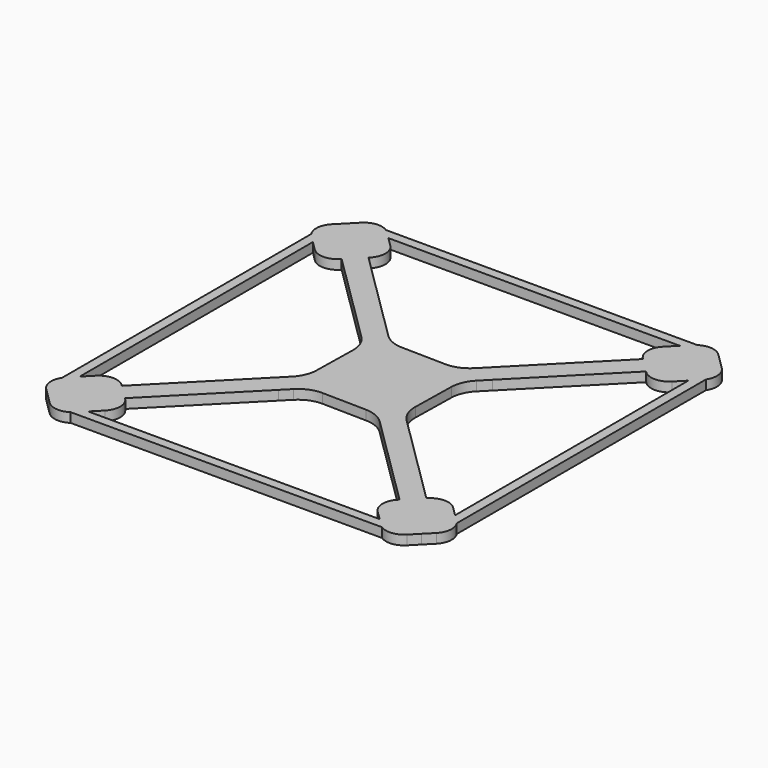
from build123d import *

# Parameters (mm, degrees)
F1_DEPTH = 4
F3_DEPTH = 4


with BuildPart() as f1:
    # F0 (on Top) → F1 (new body)
    with BuildSketch(Plane.XY):
        with BuildLine():
            Line((-64.135030253, 57.8487346722), (-60.9918824626, 60.9918824626))
            Line((-60.9918824626, 60.9918824626), (-57.8872043507, 64.1730347516))
            Line((-57.8872043507, 64.1730347516), (-57.5279368508, 64.536699731))
            ThreePointArc((-57.5279368508, 64.536699731), (-55.3289064598, 69.9383294266), (-57.5934861455, 75.3128077153))
            Line((-57.5934861455, 75.3128077153), (-61.0650929383, 78.7424354322))
            Line((-61.0650929383, 78.7424354322), (-64.536699731, 82.1720631491))
            ThreePointArc((-64.536699731, 82.1720631491), (-69.9383294266, 84.3710935402), (-75.3128077153, 82.1065138545))
            Line((-75.3128077153, 82.1065138545), (-78.7424354322, 78.6349070617))
            Line((-78.7424354322, 78.6349070617), (-82.1720631491, 75.163300269))
            ThreePointArc((-82.1720631491, 75.163300269), (-84.3710935402, 69.7616705734), (-82.1065138545, 64.3871922846))
            Line((-82.1065138545, 64.3871922846), (-75.163300269, 57.5279368508))
            ThreePointArc((-75.163300269, 57.5279368508), (-69.7616705734, 55.3289064598), (-64.3871922846, 57.5934861455))
            Line((-64.3871922846, 57.5934861455), (-64.135030253, 57.8487346722))
        make_face()
        with BuildLine():
            Line((-60.9918824626, 60.9918824626), (-24.9487193947, 24.9487193947))
            ThreePointArc((-24.9487193947, 24.9487193947), (-23.2982405477, 26.6622275187), (-21.7131078047, 28.4363596169))
            Line((-21.7131078047, 28.4363596169), (-57.8872043507, 64.1730347516))
            Line((-57.8872043507, 64.1730347516), (-60.9918824626, 60.9918824626))
        make_face()
        with BuildLine():
            ThreePointArc((-27.9685415263, 22.1195753621), (-26.4355788417, 23.5095421312), (-24.9487193947, 24.9487193947))
            Line((-24.9487193947, 24.9487193947), (-60.9918824626, 60.9918824626))
            Line((-60.9918824626, 60.9918824626), (-64.135030253, 57.8487346722))
            Line((-64.135030253, 57.8487346722), (-27.9685415263, 22.1195753621))
        make_face()
        with BuildLine():
            Line((-24.9487193947, 24.9487193947), (0, 0))
            Line((0, 0), (24.9487193947, 24.9487193947))
            ThreePointArc((24.9487193947, 24.9487193947), (23.5095421312, 26.4355788417), (22.1195753621, 27.9685415263))
            Line((22.1195753621, 27.9685415263), (18.6042693789, 24.4102077544))
            ThreePointArc((18.6042693789, 24.4102077544), (14.3526979396, 21.5708297932), (9.3259920152, 20.6380090919))
            Line((9.3259920152, 20.6380090919), (-9.2049935755, 20.9934651587))
            ThreePointArc((-9.2049935755, 20.9934651587), (-13.8982384325, 21.9899359298), (-17.8868961856, 24.6564149968))
            Line((-17.8868961856, 24.6564149968), (-21.7131078047, 28.4363596169))
            ThreePointArc((-21.7131078047, 28.4363596169), (-23.2982405477, 26.6622275187), (-24.9487193947, 24.9487193947))
        make_face()
        with BuildLine():
            Line((-24.6564149968, -17.8868961856), (-28.4363596169, -21.7131078047))
            ThreePointArc((-28.4363596169, -21.7131078047), (-26.6622275187, -23.2982405478), (-24.9487193947, -24.9487193947))
            Line((-24.9487193947, -24.9487193947), (0, 0))
            Line((0, 0), (-24.9487193947, 24.9487193947))
            ThreePointArc((-24.9487193947, 24.9487193947), (-26.4355788417, 23.5095421312), (-27.9685415263, 22.1195753621))
            Line((-27.9685415263, 22.1195753621), (-24.4102077544, 18.6042693789))
            ThreePointArc((-24.4102077544, 18.6042693789), (-21.5708297932, 14.3526979396), (-20.6380090919, 9.3259920152))
            Line((-20.6380090919, 9.3259920152), (-20.9934651587, -9.2049935755))
            ThreePointArc((-20.9934651587, -9.2049935755), (-21.9899359298, -13.8982384325), (-24.6564149968, -17.8868961856))
        make_face()
        with BuildLine():
            ThreePointArc((-24.9487193947, -24.9487193947), (-23.5095421312, -26.4355788418), (-22.1195753621, -27.9685415263))
            Line((-22.1195753621, -27.9685415263), (-18.6042693789, -24.4102077545))
            ThreePointArc((-18.6042693789, -24.4102077545), (-14.3526979396, -21.5708297932), (-9.3259920152, -20.6380090919))
            Line((-9.3259920152, -20.6380090919), (9.2049935755, -20.9934651587))
            ThreePointArc((9.2049935755, -20.9934651587), (13.8982384325, -21.9899359298), (17.8868961856, -24.6564149968))
            Line((17.8868961856, -24.6564149968), (21.7131078047, -28.4363596169))
            ThreePointArc((21.7131078047, -28.4363596169), (23.2982405477, -26.6622275187), (24.9487193947, -24.9487193947))
            Line((24.9487193947, -24.9487193947), (0, 0))
            Line((0, 0), (-24.9487193947, -24.9487193947))
        make_face()
        with BuildLine():
            Line((24.9487193947, 24.9487193947), (0, 0))
            Line((0, 0), (24.9487193947, -24.9487193947))
            ThreePointArc((24.9487193947, -24.9487193947), (26.4355788417, -23.5095421312), (27.9685415263, -22.1195753621))
            Line((27.9685415263, -22.1195753621), (24.4102077545, -18.6042693789))
            ThreePointArc((24.4102077545, -18.6042693789), (21.5708297932, -14.3526979396), (20.6380090919, -9.3259920152))
            Line((20.6380090919, -9.3259920152), (20.9934651587, 9.2049935755))
            ThreePointArc((20.9934651587, 9.2049935755), (21.9899359298, 13.8982384325), (24.6564149968, 17.8868961856))
            Line((24.6564149968, 17.8868961856), (28.4363596169, 21.7131078047))
            ThreePointArc((28.4363596169, 21.7131078047), (26.6622275187, 23.2982405477), (24.9487193947, 24.9487193947))
        make_face()
        with BuildLine():
            Line((60.9918824626, 60.9918824626), (24.9487193947, 24.9487193947))
            ThreePointArc((24.9487193947, 24.9487193947), (26.6622275187, 23.2982405477), (28.4363596169, 21.7131078047))
            Line((28.4363596169, 21.7131078047), (64.1730347516, 57.8872043507))
            Line((64.1730347516, 57.8872043507), (60.9918824626, 60.9918824626))
        make_face()
        with BuildLine():
            ThreePointArc((22.1195753621, 27.9685415263), (23.5095421312, 26.4355788417), (24.9487193947, 24.9487193947))
            Line((24.9487193947, 24.9487193947), (60.9918824626, 60.9918824626))
            Line((60.9918824626, 60.9918824626), (57.8487346722, 64.135030253))
            Line((57.8487346722, 64.135030253), (22.1195753621, 27.9685415263))
        make_face()
        with BuildLine():
            Line((57.8487346722, 64.135030253), (60.9918824626, 60.9918824626))
            Line((60.9918824626, 60.9918824626), (64.1730347516, 57.8872043507))
            Line((64.1730347516, 57.8872043507), (64.536699731, 57.5279368508))
            ThreePointArc((64.536699731, 57.5279368508), (69.9383294266, 55.3289064598), (75.3128077154, 57.5934861455))
            Line((75.3128077154, 57.5934861455), (78.7424354323, 61.0650929383))
            Line((78.7424354323, 61.0650929383), (82.1720631492, 64.536699731))
            ThreePointArc((82.1720631492, 64.536699731), (84.3710935402, 69.9383294266), (82.1065138545, 75.3128077153))
            Line((82.1065138545, 75.3128077153), (78.6349070617, 78.7424354322))
            Line((78.6349070617, 78.7424354322), (75.163300269, 82.1720631491))
            ThreePointArc((75.163300269, 82.1720631491), (69.7616705734, 84.3710935402), (64.3871922846, 82.1065138545))
            Line((64.3871922846, 82.1065138545), (57.5279368508, 75.163300269))
            ThreePointArc((57.5279368508, 75.163300269), (55.3289064598, 69.7616705734), (57.5934861455, 64.3871922846))
            Line((57.5934861455, 64.3871922846), (57.8487346722, 64.135030253))
        make_face()
        with BuildLine():
            Line((64.135030253, -57.8487346722), (60.9918824626, -60.9918824626))
            Line((60.9918824626, -60.9918824626), (57.8872043507, -64.1730347516))
            Line((57.8872043507, -64.1730347516), (57.5279368509, -64.536699731))
            ThreePointArc((57.5279368509, -64.536699731), (55.3289064598, -69.9383294266), (57.5934861455, -75.3128077154))
            Line((57.5934861455, -75.3128077154), (61.0650929383, -78.7424354323))
            Line((61.0650929383, -78.7424354323), (64.536699731, -82.1720631492))
            ThreePointArc((64.536699731, -82.1720631492), (69.9383294266, -84.3710935402), (75.3128077154, -82.1065138545))
            Line((75.3128077154, -82.1065138545), (78.7424354323, -78.6349070617))
            Line((78.7424354323, -78.6349070617), (82.1720631492, -75.163300269))
            ThreePointArc((82.1720631492, -75.163300269), (84.3710935402, -69.7616705734), (82.1065138545, -64.3871922846))
            Line((82.1065138545, -64.3871922846), (75.163300269, -57.5279368508))
            ThreePointArc((75.163300269, -57.5279368508), (69.7616705734, -55.3289064598), (64.3871922847, -57.5934861455))
            Line((64.3871922847, -57.5934861455), (64.135030253, -57.8487346722))
        make_face()
        with BuildLine():
            ThreePointArc((27.9685415263, -22.1195753621), (26.4355788417, -23.5095421312), (24.9487193947, -24.9487193947))
            Line((24.9487193947, -24.9487193947), (60.9918824626, -60.9918824626))
            Line((60.9918824626, -60.9918824626), (64.135030253, -57.8487346722))
            Line((64.135030253, -57.8487346722), (27.9685415263, -22.1195753621))
        make_face()
        with BuildLine():
            Line((60.9918824626, -60.9918824626), (24.9487193947, -24.9487193947))
            ThreePointArc((24.9487193947, -24.9487193947), (23.2982405477, -26.6622275187), (21.7131078047, -28.4363596169))
            Line((21.7131078047, -28.4363596169), (57.8872043507, -64.1730347516))
            Line((57.8872043507, -64.1730347516), (60.9918824626, -60.9918824626))
        make_face()
        with BuildLine():
            Line((-57.8487346722, -64.135030253), (-22.1195753621, -27.9685415263))
            ThreePointArc((-22.1195753621, -27.9685415263), (-23.5095421312, -26.4355788418), (-24.9487193947, -24.9487193947))
            Line((-24.9487193947, -24.9487193947), (-60.9918824626, -60.9918824626))
            Line((-60.9918824626, -60.9918824626), (-57.8487346722, -64.135030253))
        make_face()
        with BuildLine():
            ThreePointArc((-24.9487193947, -24.9487193947), (-26.6622275187, -23.2982405478), (-28.4363596169, -21.7131078047))
            Line((-28.4363596169, -21.7131078047), (-64.1730347516, -57.8872043507))
            Line((-64.1730347516, -57.8872043507), (-60.9918824626, -60.9918824626))
            Line((-60.9918824626, -60.9918824626), (-24.9487193947, -24.9487193947))
        make_face()
        with BuildLine():
            Line((-57.5934861455, -64.3871922847), (-57.8487346722, -64.135030253))
            Line((-57.8487346722, -64.135030253), (-60.9918824626, -60.9918824626))
            Line((-60.9918824626, -60.9918824626), (-64.1730347516, -57.8872043507))
            Line((-64.1730347516, -57.8872043507), (-64.536699731, -57.5279368509))
            ThreePointArc((-64.536699731, -57.5279368509), (-69.9383294266, -55.3289064598), (-75.3128077153, -57.5934861455))
            Line((-75.3128077153, -57.5934861455), (-78.7424354322, -61.0650929383))
            Line((-78.7424354322, -61.0650929383), (-82.1720631491, -64.536699731))
            ThreePointArc((-82.1720631491, -64.536699731), (-84.3710935402, -69.9383294266), (-82.1065138545, -75.3128077154))
            Line((-82.1065138545, -75.3128077154), (-78.6349070617, -78.7424354323))
            Line((-78.6349070617, -78.7424354323), (-75.163300269, -82.1720631492))
            ThreePointArc((-75.163300269, -82.1720631492), (-69.7616705734, -84.3710935402), (-64.3871922846, -82.1065138545))
            Line((-64.3871922846, -82.1065138545), (-57.5279368508, -75.163300269))
            ThreePointArc((-57.5279368508, -75.163300269), (-55.3289064598, -69.7616705734), (-57.5934861455, -64.3871922847))
        make_face()
    extrude(amount=F1_DEPTH)

    # F2 (on face) → F3 (join)
    with BuildSketch(Plane.XY.offset(4)):
        with BuildLine():
            ThreePointArc((-64.3871922846, -82.1065138545), (-64.9658566006, -82.634927624), (-65.5957303462, -83.1011170351))
            Line((-65.5957303462, -83.1011170351), (65.6796884979, -83.1011170351))
            ThreePointArc((65.6796884979, -83.1011170351), (65.0856932086, -82.6642723213), (64.536699731, -82.1720631492))
            Line((64.536699731, -82.1720631492), (61.4281648492, -79.1011170351))
            Line((61.4281648492, -79.1011170351), (-61.4181370755, -79.1011170351))
            Line((-61.4181370755, -79.1011170351), (-64.3871922846, -82.1065138545))
        make_face()
        with BuildLine():
            ThreePointArc((-75.163300269, -82.1720631492), (-70.5444929949, -84.335561038), (-65.5957303462, -83.1011170351))
            ThreePointArc((-65.5957303462, -83.1011170351), (-64.9658566006, -82.634927624), (-64.3871922846, -82.1065138545))
            Line((-64.3871922846, -82.1065138545), (-61.4181370755, -79.1011170351))
            Line((-61.4181370755, -79.1011170351), (-57.5279368508, -75.163300269))
            ThreePointArc((-57.5279368508, -75.163300269), (-55.3289064598, -69.7616705734), (-57.5934861455, -64.3871922847))
            Line((-57.5934861455, -64.3871922847), (-57.8487346722, -64.135030253))
            Line((-57.8487346722, -64.135030253), (-18.6042693789, -24.4102077545))
            ThreePointArc((-18.6042693789, -24.4102077545), (-14.3526979396, -21.5708297932), (-9.3259920152, -20.6380090919))
            Line((-9.3259920152, -20.6380090919), (9.2049935755, -20.9934651587))
            ThreePointArc((9.2049935755, -20.9934651587), (13.8982384325, -21.9899359298), (17.8868961856, -24.6564149968))
            Line((17.8868961856, -24.6564149968), (57.8872043507, -64.1730347516))
            Line((57.8872043507, -64.1730347516), (57.5279368509, -64.536699731))
            ThreePointArc((57.5279368509, -64.536699731), (55.3289064598, -69.9383294266), (57.5934861455, -75.3128077154))
            Line((57.5934861455, -75.3128077154), (61.4281648492, -79.1011170351))
            Line((61.4281648492, -79.1011170351), (64.536699731, -82.1720631492))
            ThreePointArc((64.536699731, -82.1720631492), (65.0856932086, -82.6642723213), (65.6796884979, -83.1011170351))
            ThreePointArc((65.6796884979, -83.1011170351), (70.6745708809, -84.3309409727), (75.3128077154, -82.1065138545))
            Line((75.3128077154, -82.1065138545), (82.1720631492, -75.163300269))
            ThreePointArc((82.1720631492, -75.163300269), (84.335561038, -70.5444929949), (83.1011170351, -65.5957303462))
            ThreePointArc((83.1011170351, -65.5957303462), (82.634927624, -64.9658566006), (82.1065138545, -64.3871922846))
            Line((82.1065138545, -64.3871922846), (79.1011170351, -61.4181370755))
            Line((79.1011170351, -61.4181370755), (75.163300269, -57.5279368508))
            ThreePointArc((75.163300269, -57.5279368508), (69.7616705734, -55.3289064598), (64.3871922847, -57.5934861455))
            Line((64.3871922847, -57.5934861455), (64.135030253, -57.8487346722))
            Line((64.135030253, -57.8487346722), (24.4102077545, -18.6042693789))
            ThreePointArc((24.4102077545, -18.6042693789), (21.5708297932, -14.3526979396), (20.6380090919, -9.3259920152))
            Line((20.6380090919, -9.3259920152), (20.9934651587, 9.2049935755))
            ThreePointArc((20.9934651587, 9.2049935755), (21.9899359298, 13.8982384325), (24.6564149968, 17.8868961856))
            Line((24.6564149968, 17.8868961856), (64.1730347516, 57.8872043507))
            Line((64.1730347516, 57.8872043507), (64.536699731, 57.5279368508))
            ThreePointArc((64.536699731, 57.5279368508), (69.9383294266, 55.3289064598), (75.3128077154, 57.5934861455))
            Line((75.3128077154, 57.5934861455), (79.1011170351, 61.4281648492))
            Line((79.1011170351, 61.4281648492), (82.1720631492, 64.536699731))
            ThreePointArc((82.1720631492, 64.536699731), (82.6642723213, 65.0856932086), (83.1011170351, 65.6796884979))
            ThreePointArc((83.1011170351, 65.6796884979), (84.3309409727, 70.6745708809), (82.1065138545, 75.3128077153))
            Line((82.1065138545, 75.3128077153), (75.163300269, 82.1720631491))
            ThreePointArc((75.163300269, 82.1720631491), (70.5444929949, 84.335561038), (65.5957303462, 83.1011170351))
            ThreePointArc((65.5957303462, 83.1011170351), (64.9658566006, 82.634927624), (64.3871922846, 82.1065138545))
            Line((64.3871922846, 82.1065138545), (61.4181370755, 79.1011170351))
            Line((61.4181370755, 79.1011170351), (57.5279368508, 75.163300269))
            ThreePointArc((57.5279368508, 75.163300269), (55.3289064598, 69.7616705734), (57.5934861455, 64.3871922846))
            Line((57.5934861455, 64.3871922846), (57.8487346722, 64.135030253))
            Line((57.8487346722, 64.135030253), (18.6042693789, 24.4102077544))
            ThreePointArc((18.6042693789, 24.4102077544), (14.3526979396, 21.5708297932), (9.3259920152, 20.6380090919))
            Line((9.3259920152, 20.6380090919), (-9.2049935755, 20.9934651587))
            ThreePointArc((-9.2049935755, 20.9934651587), (-13.8982384325, 21.9899359298), (-17.8868961856, 24.6564149968))
            Line((-17.8868961856, 24.6564149968), (-57.8872043507, 64.1730347516))
            Line((-57.8872043507, 64.1730347516), (-57.5279368508, 64.536699731))
            ThreePointArc((-57.5279368508, 64.536699731), (-55.3289064598, 69.9383294266), (-57.5934861455, 75.3128077153))
            Line((-57.5934861455, 75.3128077153), (-61.4281648492, 79.1011170351))
            Line((-61.4281648492, 79.1011170351), (-64.536699731, 82.1720631491))
            ThreePointArc((-64.536699731, 82.1720631491), (-65.0856932086, 82.6642723213), (-65.6796884979, 83.1011170351))
            ThreePointArc((-65.6796884979, 83.1011170351), (-70.6745708809, 84.3309409727), (-75.3128077153, 82.1065138545))
            Line((-75.3128077153, 82.1065138545), (-82.1720631491, 75.163300269))
            ThreePointArc((-82.1720631491, 75.163300269), (-84.335561038, 70.5444929949), (-83.1011170351, 65.5957303462))
            ThreePointArc((-83.1011170351, 65.5957303462), (-82.634927624, 64.9658566006), (-82.1065138545, 64.3871922846))
            Line((-82.1065138545, 64.3871922846), (-79.1011170351, 61.4181370755))
            Line((-79.1011170351, 61.4181370755), (-75.163300269, 57.5279368508))
            ThreePointArc((-75.163300269, 57.5279368508), (-69.7616705734, 55.3289064598), (-64.3871922846, 57.5934861455))
            Line((-64.3871922846, 57.5934861455), (-64.135030253, 57.8487346722))
            Line((-64.135030253, 57.8487346722), (-24.4102077544, 18.6042693789))
            ThreePointArc((-24.4102077544, 18.6042693789), (-21.5708297932, 14.3526979396), (-20.6380090919, 9.3259920152))
            Line((-20.6380090919, 9.3259920152), (-20.9934651587, -9.2049935755))
            ThreePointArc((-20.9934651587, -9.2049935755), (-21.9899359298, -13.8982384325), (-24.6564149968, -17.8868961856))
            Line((-24.6564149968, -17.8868961856), (-64.1730347516, -57.8872043507))
            Line((-64.1730347516, -57.8872043507), (-64.536699731, -57.5279368509))
            ThreePointArc((-64.536699731, -57.5279368509), (-69.9383294266, -55.3289064598), (-75.3128077153, -57.5934861455))
            Line((-75.3128077153, -57.5934861455), (-79.1011170351, -61.4281648492))
            Line((-79.1011170351, -61.4281648492), (-82.1720631491, -64.536699731))
            ThreePointArc((-82.1720631491, -64.536699731), (-82.6642723213, -65.0856932086), (-83.1011170351, -65.6796884979))
            ThreePointArc((-83.1011170351, -65.6796884979), (-84.3309409727, -70.6745708809), (-82.1065138545, -75.3128077154))
            Line((-82.1065138545, -75.3128077154), (-75.163300269, -82.1720631492))
        make_face()
        with BuildLine():
            Line((-83.1011170351, 65.5957303462), (-83.1011170351, -65.6796884979))
            ThreePointArc((-83.1011170351, -65.6796884979), (-82.6642723213, -65.0856932086), (-82.1720631491, -64.536699731))
            Line((-82.1720631491, -64.536699731), (-79.1011170351, -61.4281648492))
            Line((-79.1011170351, -61.4281648492), (-79.1011170351, 61.4181370755))
            Line((-79.1011170351, 61.4181370755), (-82.1065138545, 64.3871922846))
            ThreePointArc((-82.1065138545, 64.3871922846), (-82.634927624, 64.9658566006), (-83.1011170351, 65.5957303462))
        make_face()
        with BuildLine():
            ThreePointArc((82.1065138545, -64.3871922846), (82.634927624, -64.9658566006), (83.1011170351, -65.5957303462))
            Line((83.1011170351, -65.5957303462), (83.1011170351, 65.6796884979))
            ThreePointArc((83.1011170351, 65.6796884979), (82.6642723213, 65.0856932086), (82.1720631492, 64.536699731))
            Line((82.1720631492, 64.536699731), (79.1011170351, 61.4281648492))
            Line((79.1011170351, 61.4281648492), (79.1011170351, -61.4181370755))
            Line((79.1011170351, -61.4181370755), (82.1065138545, -64.3871922846))
        make_face()
        with BuildLine():
            Line((65.5957303462, 83.1011170351), (-65.6796884979, 83.1011170351))
            ThreePointArc((-65.6796884979, 83.1011170351), (-65.0856932086, 82.6642723213), (-64.536699731, 82.1720631491))
            Line((-64.536699731, 82.1720631491), (-61.4281648492, 79.1011170351))
            Line((-61.4281648492, 79.1011170351), (61.4181370755, 79.1011170351))
            Line((61.4181370755, 79.1011170351), (64.3871922846, 82.1065138545))
            ThreePointArc((64.3871922846, 82.1065138545), (64.9658566006, 82.634927624), (65.5957303462, 83.1011170351))
        make_face()
    extrude(amount=-F3_DEPTH)


solid = f1.part
